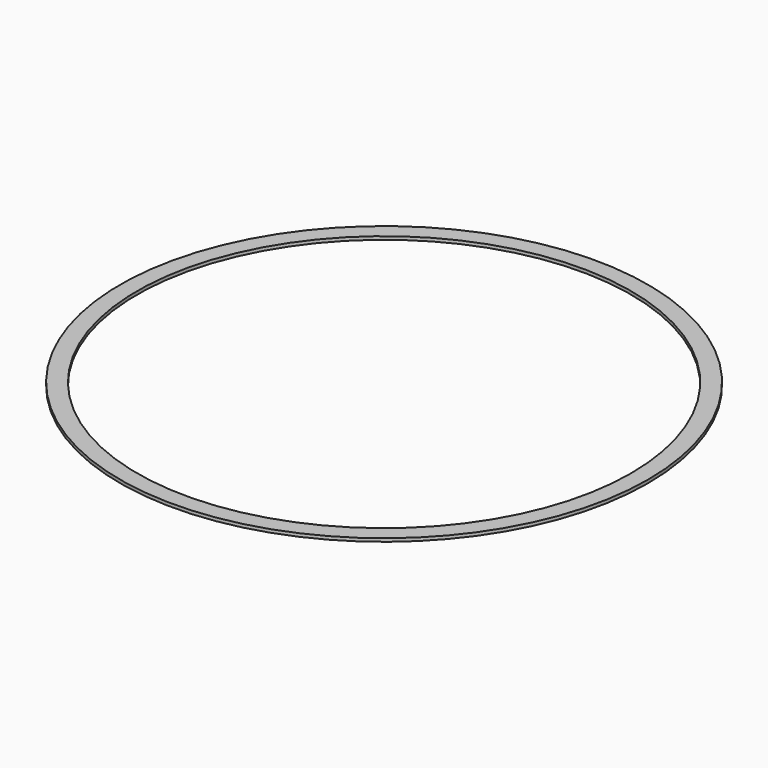
from build123d import *

# Parameters (mm, degrees)
F0_R     = 393.09802
F0_R_2   = 367.69802
F1_DEPTH = 4.7625


# Not quite as in the source:
# - a length typed as a fraction of an inch, garbled in the dataset ("3 / 203.2 mm" for 3/8 in), is restored


with BuildPart() as f1:
    # F0 (on Top) → F1 (new body)
    with BuildSketch(Plane.XY):
        Circle(F0_R)
        Circle(F0_R_2, mode=Mode.SUBTRACT)
    extrude(amount=F1_DEPTH)


solid = f1.part
